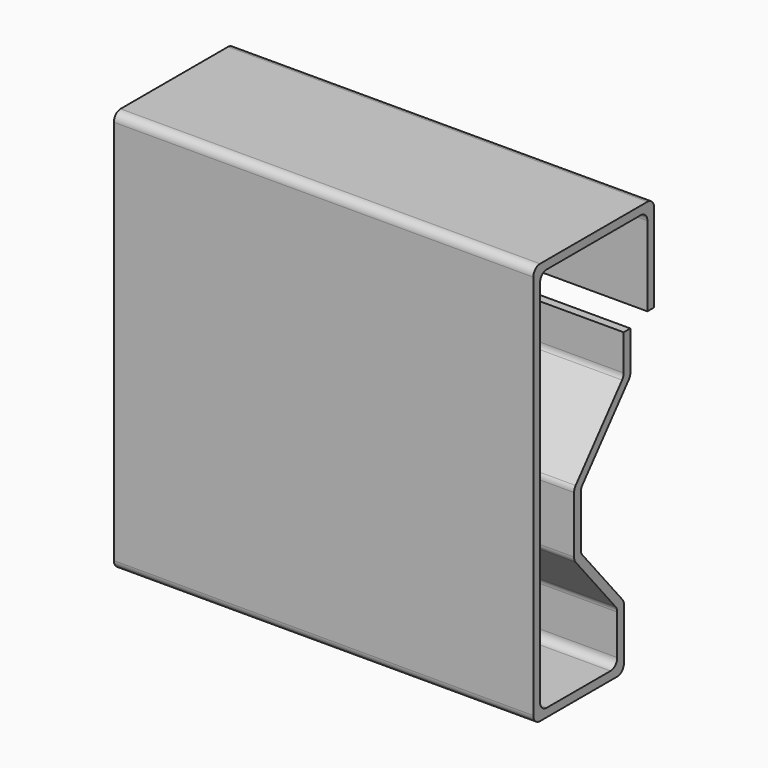
from build123d import *

# Parameters (mm, degrees)
F1_DEPTH = 100
F2_R     = 2


with BuildPart() as f1:
    # F0 (on Right) → F1 (new body)
    with BuildSketch(Plane.YZ):
        Polygon((34, -23), (36, -23), (36, 0), (0, 0), (0, -96), (27, -96), (27, -81), (14.1442478063, -65.6791111376), (14.1442478063, -52.1349920747), (28.9283628291, -34.5159698829), (28.9283628291, -24.5159698829), (26.9283628291, -24.5159698829), (26.9283628291, -33.7880294144), (12.1442478063, -51.4070516062), (12.1442478063, -66.4070516062), (25, -81.7279404685), (25, -94), (2, -94), (2, -2), (34, -2), align=None)
    extrude(amount=F1_DEPTH)

    # F2
    f2_edges = [f1.edges().sort_by_distance(p)[0] for p in [
        (50, 36, 0),
        (50, 0, 0),
        (50, 34, -2),
        (50, 2, -2),
        (50, 0, -96),
        (50, 27, -96),
        (50, 27, -81),
        (50, 28.928363, -34.51597),
        (50, 2, -94),
        (50, 25, -94),
        (50, 25, -81.72794),
        (50, 26.928363, -33.788029),
        (50, 14.144248, -65.679111),
        (50, 14.144248, -52.134992),
        (50, 12.144248, -51.407052),
        (50, 12.144248, -66.407052),
    ]]
    fillet(f2_edges, radius=F2_R)


solid = f1.part
